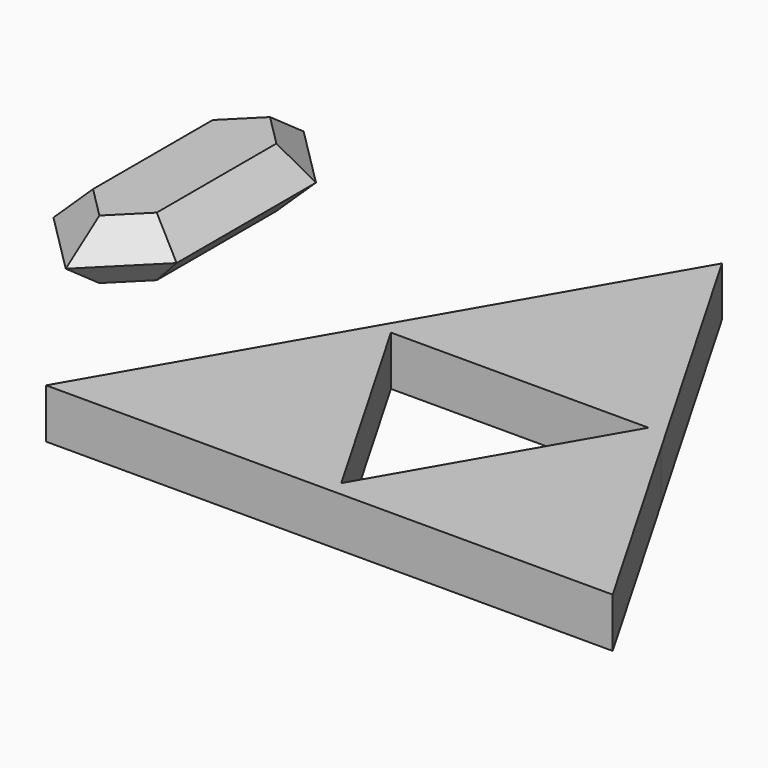
from build123d import *

# Parameters (mm, degrees)
F1_DEPTH = 6
F2_SIZE  = 2.99999
F4_DEPTH = 5


# Not quite as in the source:
# - a fillet or chamfer is up to 0.001 mm smaller than in the source, because OpenCascade refuses the exact size


with BuildPart() as f1:
    # F0 (on Top) → F1 (new body)
    with BuildSketch(Plane.XY):
        Polygon((-6.2132034356, 8.7867965644), (-6.2132034356, 0), (-6.2132034356, -8.7867965644), (0, -15), (6.2132034356, -8.7867965644), (6.2132034356, 0), (6.2132034356, 8.7867965644), (0, 15), align=None)
    extrude(amount=F1_DEPTH)

    # F2 (size 3 in the source; OpenCascade refuses exactly that, so slightly less here)
    f2_edges = [f1.edges().sort_by_distance(p)[0] for p in [
        (-3.106602, 11.893398, 6),
        (3.106602, 11.893398, 6),
        (6.213203, 0, 6),
        (-6.213203, 0, 6),
        (-3.106602, -11.893398, 6),
        (3.106602, -11.893398, 6),
        (-3.106602, 11.893398, 0),
        (-6.213203, 0, 0),
        (-3.106602, -11.893398, 0),
        (3.106602, -11.893398, 0),
        (6.213203, 0, 0),
        (3.106602, 11.893398, 0),
    ]]
    chamfer(f2_edges, length=F2_SIZE)


with BuildPart() as f4:
    # F3 (on Top) → F4 (new body)
    with BuildSketch(Plane.XY):
        Polygon((28.300814713, -9.0636431253), (13.6151272242, -34.5), (28.8406131639, -34.5), (70.772803874, -34.5), (58.1850934371, -12.6974459723), (42.1939655491, 15), align=None)
        Polygon((29.2035844924, -10.5), (42.1939655491, -10.5), (55.1843466059, -10.5), (42.1939655491, -33), align=None, mode=Mode.SUBTRACT)
    extrude(amount=F4_DEPTH)


solid = Compound([f1.part, f4.part])
